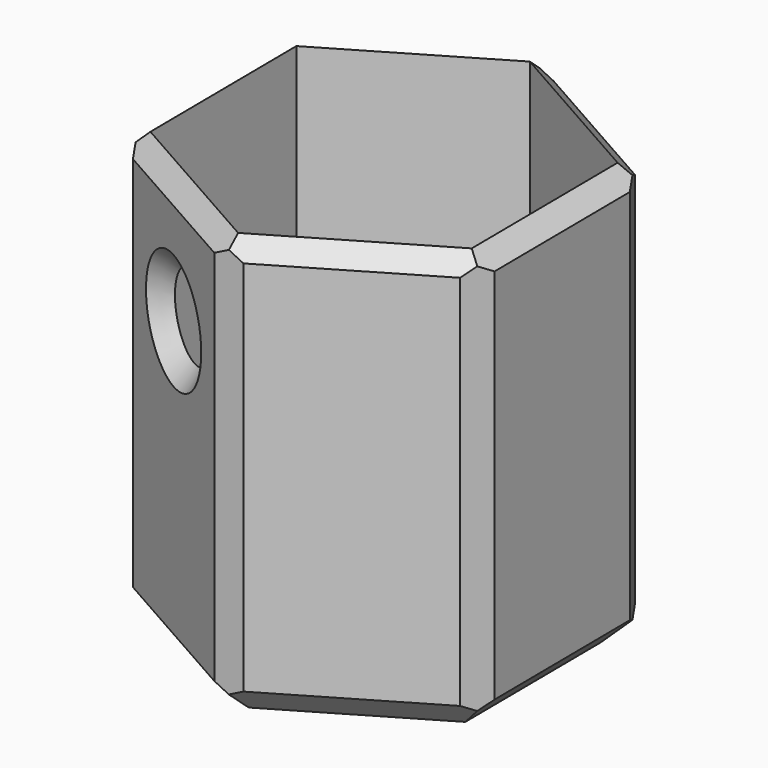
from build123d import *

# Parameters (mm, degrees)
F1_DEPTH     = 75
F2_T         = -3
F3_SIZE      = 5
F4_T1_DEPTH  = 60.9562282093
F4_T3_DEPTH  = 60.9562282093
F4_T5_DEPTH  = 60.9562282093
F4_T7_DEPTH  = 60.9562282093
F4_T9_DEPTH  = 60.9562282093
F4_T11_DEPTH = 60.9562282093
F6_D         = 10
F7_T1_DEPTH  = 80.3079500043


# Not quite as in the source:
# - a fillet or chamfer that OpenCascade refuses, or shapes differently, is made with other operations: its cross-section is extruded or revolved along the edge and cut away or added


with BuildPart() as f1:
    # F0 (on Top) → F1 (new body)
    with BuildSketch(Plane.XY):
        Polygon((-0.2972451442, 35.2381446725), (-30.6657510407, 17.3616504902), (-30.3685058965, -17.8764941822), (0.2972451442, -35.2381446725), (30.6657510407, -17.3616504902), (30.3685058965, 17.8764941822), align=None)
    extrude(amount=F1_DEPTH)

    # F2
    f2_openings = [f1.faces().sort_by_distance(p)[0] for p in [
        (0, 0, 75),
    ]]
    offset(amount=F2_T, openings=f2_openings)

    # F3
    f3_edges = [f1.edges().sort_by_distance(p)[0] for p in [
        (15.03563, 26.557319, 0),
        (-15.481498, 26.299898, 0),
        (-30.517128, -0.257422, 0),
        (-15.03563, -26.557319, 0),
        (15.481498, -26.299898, 0),
        (30.517128, 0.257422, 0),
    ]]
    chamfer(f3_edges, length=F3_SIZE)

    # F4: chamfer of 5 on 6 edges, made by hand

    # F4_s2 → F4_t1 (cut)
    with BuildSketch(Plane(origin=(-26.5224238672, 15.0158739867, 0), x_dir=(0, 0, 1), z_dir=(0.8702121062, -0.4926772679, 0))):
        Polygon((75, 25.5182141675), (70, 30.5182141675), (75, 30.5182141675), align=None)
    extrude(amount=F4_T1_DEPTH, mode=Mode.SUBTRACT)

    # F4_s4 → F4_t3 (cut)
    with BuildSketch(Plane(origin=(-0.257083601, 30.4770298323, 0), x_dir=(0, 0, 1), z_dir=(0.0084350232, -0.9999644246, 0))):
        Polygon((75, 25.5182141675), (70, 30.5182141675), (75, 30.5182141675), align=None)
    extrude(amount=F4_T3_DEPTH, mode=Mode.SUBTRACT)

    # F4_s6 → F4_t5 (cut)
    with BuildSketch(Plane(origin=(26.2653402661, 15.4611558455, 0), x_dir=(0, 0, 1), z_dir=(-0.8617770829, -0.5072871567, 0))):
        Polygon((75, 25.5182141675), (70, 30.5182141675), (75, 30.5182141675), align=None)
    extrude(amount=F4_T5_DEPTH, mode=Mode.SUBTRACT)

    # F4_s8 → F4_t7 (cut)
    with BuildSketch(Plane(origin=(26.5224238672, -15.0158739867, 0), x_dir=(0, 0, 1), z_dir=(-0.8702121062, 0.4926772679, 0))):
        Polygon((70, 30.5182141675), (75, 25.5182141675), (75, 30.5182141675), align=None)
    extrude(amount=F4_T7_DEPTH, mode=Mode.SUBTRACT)

    # F4_s10 → F4_t9 (cut)
    with BuildSketch(Plane(origin=(0.257083601, -30.4770298323, 0), x_dir=(0, 0, 1), z_dir=(-0.0084350232, 0.9999644246, 0))):
        Polygon((70, 30.5182141675), (75, 25.5182141675), (75, 30.5182141675), align=None)
    extrude(amount=F4_T9_DEPTH, mode=Mode.SUBTRACT)

    # F4_s12 → F4_t11 (cut)
    with BuildSketch(Plane(origin=(-26.2653402661, -15.4611558455, 0), x_dir=(0, 0, 1), z_dir=(0.8617770829, 0.5072871567, 0))):
        Polygon((75, 25.5182141675), (70, 30.5182141675), (75, 30.5182141675), align=None)
    extrude(amount=F4_T11_DEPTH, mode=Mode.SUBTRACT)

    # F6 (through all)
    with Locations(Plane(origin=(-15.0356303762, -26.5573194273, 0), x_dir=(0.8702121062, -0.4926772679, 0), z_dir=(-0.4926772679, -0.8702121062, 0))):
        with Locations((0, 52.5516085327)):
            Hole(F6_D / 2)

    # F7: chamfer of 5 on 8 edges, made by hand

    # F7_s2 → F7_t1 (cut)
    with BuildSketch(Plane.XY.offset(-2.6539750021)):
        Polygon((-30.3928557112, -14.9898455337), (-27.8564199277, -19.2987309484), (-30.3685058965, -17.8764941822), align=None)
        Polygon((-28.1780148866, 18.8260623726), (-30.6414012259, 14.4750018417), (-30.6657510407, 17.3616504902), align=None)
        Polygon((2.2148408246, 33.8159079063), (-2.7849812982, 33.7737327901), (-0.2972451442, 35.2381446725), align=None)
        Polygon((27.8564199277, 19.2987309484), (30.3928557112, 14.9898455337), (30.3685058965, 17.8764941822), align=None)
        Polygon((30.6414012259, -14.4750018417), (28.1780148866, -18.8260623726), (30.6657510407, -17.3616504902), align=None)
        Polygon((2.7849812982, -33.7737327901), (-2.2148408246, -33.8159079063), (0.2972451442, -35.2381446725), align=None)
    extrude(amount=F7_T1_DEPTH, mode=Mode.SUBTRACT)

    # F7_s3 → F7_t4 (revolve, cut)
    with BuildSketch(Plane.XY.offset(52.5516085327)):
        Polygon((23.7377514379, 21.6305467487), (16.9233045677, 19.7428725572), (19.386690907, 24.093933088), align=None)
    revolve(axis=Axis((15.0356303762, 26.5573194273, 52.5516085327), (-0.4926772679, -0.8702121062, 0)), mode=Mode.SUBTRACT)

    # F7_s5 → F7_t6 (revolve, cut)
    with BuildSketch(Plane.XY.offset(52.5516085327)):
        Polygon((-6.3335093144, -31.484092106), (-8.221183506, -24.6696452358), (-10.6845698453, -29.0207057667), align=None)
    revolve(axis=Axis((-15.0356303762, -26.5573194273, 52.5516085327), (-0.4926772679, -0.8702121062, 0)), mode=Mode.SUBTRACT)


solid = f1.part
